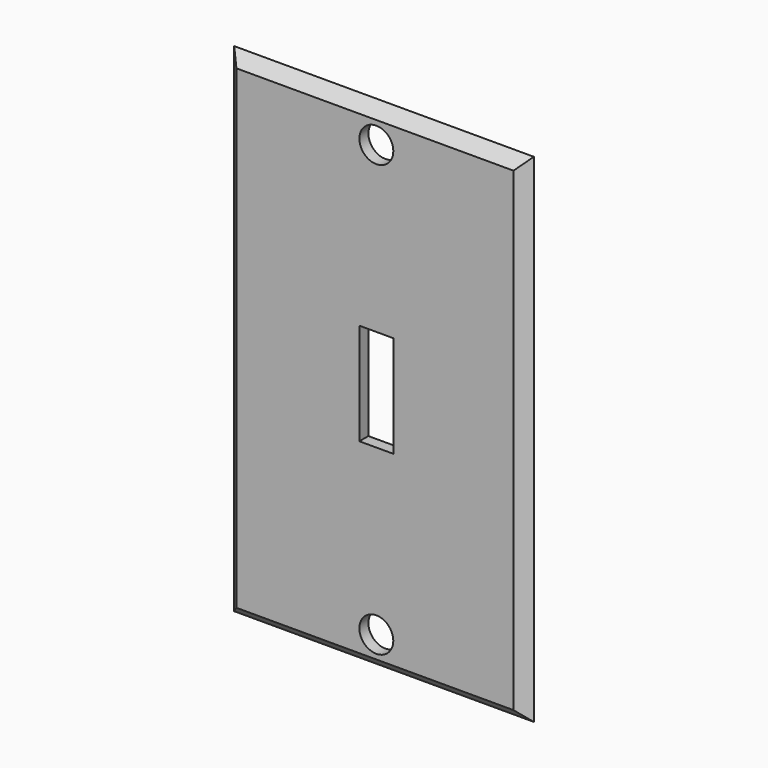
from build123d import *

# Parameters (mm, degrees)
F0_W        = 69.85
F0_H        = 114.3
F0_R        = 3.81
F1_DEPTH    = 2.54
F2_T1_DEPTH = 89.4462243683
F2_T3_DEPTH = 133.8962243683


# Not quite as in the source:
# - a fillet or chamfer that OpenCascade refuses, or shapes differently, is made with other operations: its cross-section is extruded or revolved along the edge and cut away or added


with BuildPart() as f1:
    # F0 (on Front) → F1 (new body)
    with BuildSketch(Plane.XZ):
        with Locations((-0.3112182021, 0)):
            Rectangle(F0_W, F0_H)
        with Locations((0, -48.4124)):
            Circle(F0_R, mode=Mode.SUBTRACT)
        Polygon((-3.81, 11.43), (0, 11.43), (3.81, 11.43), (3.81, -11.43), (-3.81, -11.43), align=None, mode=Mode.SUBTRACT)
        with Locations((0, 48.4124)):
            Circle(F0_R, mode=Mode.SUBTRACT)
    extrude(amount=F1_DEPTH)

    # F2: chamfer of 3.81 on 4 edges, made by hand

    # F2_s2 → F2_t1 (cut)
    with BuildSketch(Plane.YZ.offset(-45.0343303863)):
        Polygon((-2.54, 53.34), (1.27, 57.15), (-2.54, 57.15), align=None)
        Polygon((-2.54, -53.34), (1.27, -57.15), (-2.54, -57.15), align=None)
    extrude(amount=F2_T1_DEPTH, mode=Mode.SUBTRACT)

    # F2_s4 → F2_t3 (cut)
    with BuildSketch(Plane.XY.offset(-66.9481121842)):
        Polygon((-31.4262182021, -2.54), (-35.2362182021, 1.27), (-35.2362182021, -2.54), align=None)
        Polygon((34.6137817979, 1.27), (30.8037817979, -2.54), (34.6137817979, -2.54), align=None)
    extrude(amount=F2_T3_DEPTH, mode=Mode.SUBTRACT)


solid = f1.part
